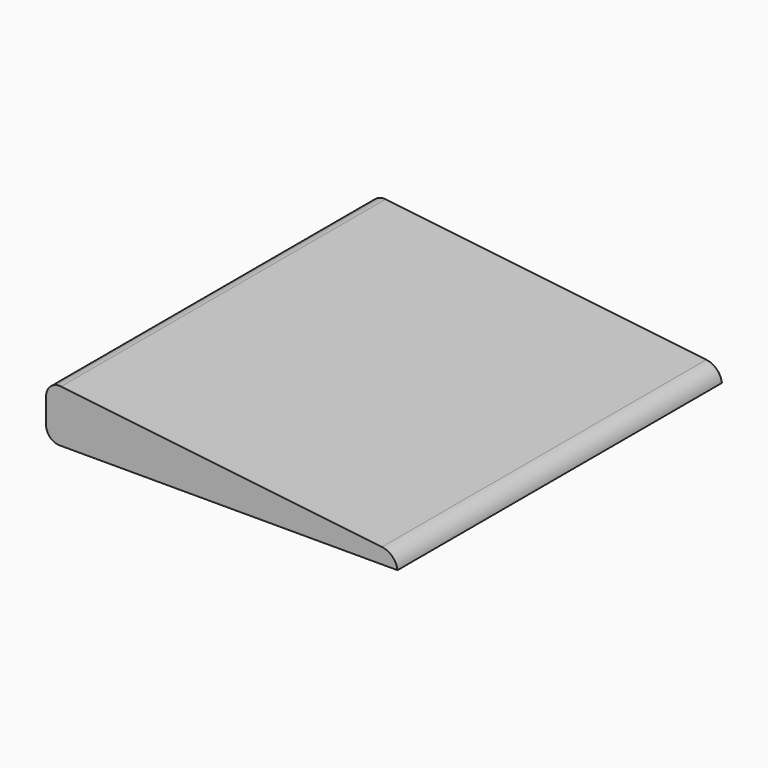
from build123d import *

# Parameters (mm, degrees)
F1_DEPTH = 150
F2_R     = 5


with BuildPart() as f1:
    # F0 (on Front) → F1 (new body)
    with BuildSketch(Plane.XZ):
        with BuildLine():
            Line((-82.3190790229, 12.2144147383), (-82.3190790229, -7.7855852617))
            Line((-82.3190790229, -7.7855852617), (47.6809209771, -7.7855852617))
            ThreePointArc((47.6809209771, -7.7855852617), (45.7765227323, -3.9495345355), (41.9135876, -2.1002779249))
            Line((41.9135876, -2.1002779249), (-82.3190790229, 12.2144147383))
        make_face()
    extrude(amount=F1_DEPTH)

    # F2
    f2_edges = [f1.edges().sort_by_distance(p)[0] for p in [
        (-82.319079, -75, 12.214415),
        (-82.319079, -75, -7.785585),
    ]]
    fillet(f2_edges, radius=F2_R)


solid = f1.part
